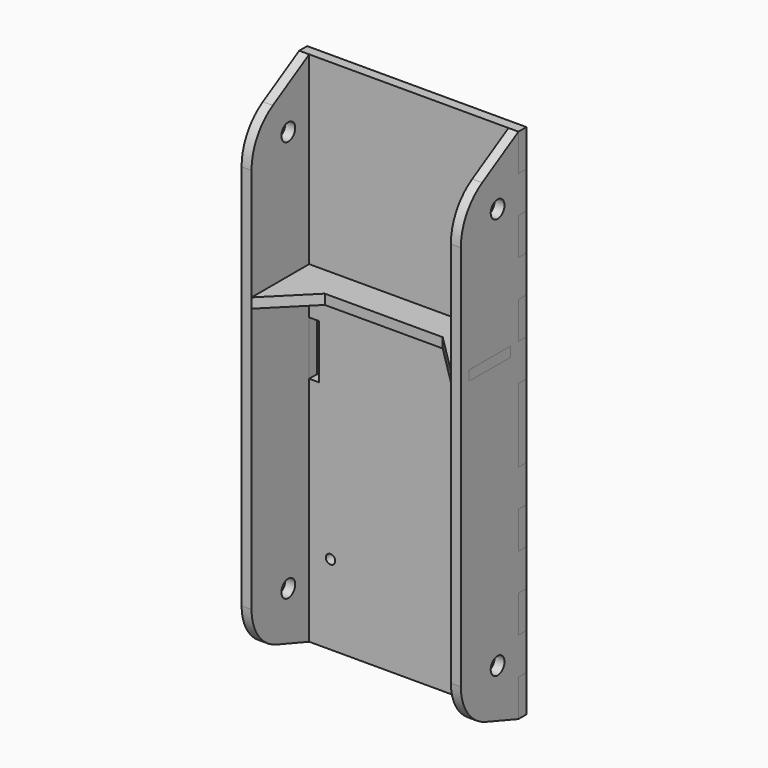
from build123d import *

# Parameters (mm, degrees)
F2_R     = 1.5
F2_W     = 3.175
F2_H     = 17.2357142857
F2_W_2   = 40
F2_H_2   = 3.175
F3_DEPTH = 3.175
F5_START = 31.825
F4_R     = 2.75
F4_W     = 16.65
F4_H     = 3.175
F5_DEPTH = 3.175
F8_DEPTH = 3.175


# Not quite as in the source:
# - a length typed as a fraction of an inch, garbled in the dataset ("3 / 203.2 mm" for 3/8 in), is restored


with BuildPart() as f3:
    # F2 (on Front) → F3 (new body)
    with BuildSketch(Plane.XZ):
        Polygon((-35, -25.4), (0, -25.4), (35, -25.4), (35, -13.6071428571), (31.825, -13.6071428571), (31.825, -1.8142857143), (35, -1.8142857143), (35, 9.9785714286), (31.825, 9.9785714286), (31.825, 21.7714285714), (35, 21.7714285714), (35, 33.5642857143), (31.825, 33.5642857143), (31.825, 45.3571428571), (35, 45.3571428571), (35, 57.15), (35, 68.9428571429), (31.825, 68.9428571429), (31.825, 80.7357142857), (35, 80.7357142857), (35, 92.5285714286), (31.825, 92.5285714286), (31.825, 104.3214285714), (35, 104.3214285714), (35, 116.1142857143), (31.825, 116.1142857143), (31.825, 127.9071428571), (35, 127.9071428571), (35, 139.7), (0, 139.7), (-35, 139.7), (-35, 127.9071428571), (-31.825, 127.9071428571), (-31.825, 116.1142857143), (-35, 116.1142857143), (-35, 104.3214285714), (-31.825, 104.3214285714), (-31.825, 92.5285714286), (-35, 92.5285714286), (-35, 80.7357142857), (-31.825, 80.7357142857), (-31.825, 68.9428571429), (-35, 68.9428571429), (-35, 57.15), (-35, 45.3571428571), (-31.825, 45.3571428571), (-31.825, 33.5642857143), (-35, 33.5642857143), (-35, 21.7714285714), (-31.825, 21.7714285714), (-31.825, 9.9785714286), (-35, 9.9785714286), (-35, -1.8142857143), (-31.825, -1.8142857143), (-31.825, -13.6071428571), (-35, -13.6071428571), align=None)
        with Locations((-25, 0)):
            Circle(F2_R, mode=Mode.SUBTRACT)
        with Locations((25, 0)):
            Circle(F2_R, mode=Mode.SUBTRACT)
        with Locations((-30.2375, 57.15)):
            Rectangle(F2_W, F2_H, mode=Mode.SUBTRACT)
        with Locations((0, 79.1482142857)):
            Rectangle(F2_W_2, F2_H_2, mode=Mode.SUBTRACT)
        with Locations((30.2375, 57.15)):
            Rectangle(F2_W, F2_H, mode=Mode.SUBTRACT)
    extrude(amount=F3_DEPTH)


with BuildPart() as f5:
    # F4 (on Right) → F5 (new body)
    with BuildSketch(Plane.YZ.offset(F5_START)):
        with BuildLine():
            Line((-16.2899039976, -20.8712812924), (-3.175, -25.4))
            Line((-3.175, -25.4), (-3.175, -13.6071428571))
            Line((-3.175, -13.6071428571), (0, -13.6071428571))
            Line((0, -13.6071428571), (0, -1.8142857143))
            Line((0, -1.8142857143), (-3.175, -1.8142857143))
            Line((-3.175, -1.8142857143), (-3.175, 9.9785714286))
            Line((-3.175, 9.9785714286), (0, 9.9785714286))
            Line((0, 9.9785714286), (0, 21.7714285714))
            Line((0, 21.7714285714), (-3.175, 21.7714285714))
            Line((-3.175, 21.7714285714), (-3.175, 33.5642857143))
            Line((-3.175, 33.5642857143), (0, 33.5642857143))
            Line((0, 33.5642857143), (0, 45.3571428571))
            Line((0, 45.3571428571), (-3.175, 45.3571428571))
            Line((-3.175, 45.3571428571), (-3.175, 57.15))
            Line((-3.175, 57.15), (-3.175, 68.9428571429))
            Line((-3.175, 68.9428571429), (0, 68.9428571429))
            Line((0, 68.9428571429), (0, 80.7357142857))
            Line((0, 80.7357142857), (-3.175, 80.7357142857))
            Line((-3.175, 80.7357142857), (-3.175, 92.5285714286))
            Line((-3.175, 92.5285714286), (0, 92.5285714286))
            Line((0, 92.5285714286), (0, 104.3214285714))
            Line((0, 104.3214285714), (-3.175, 104.3214285714))
            Line((-3.175, 104.3214285714), (-3.175, 116.1142857143))
            Line((-3.175, 116.1142857143), (0, 116.1142857143))
            Line((0, 116.1142857143), (0, 127.9071428571))
            Line((0, 127.9071428571), (-3.175, 127.9071428571))
            Line((-3.175, 127.9071428571), (-3.175, 139.7))
            Line((-3.175, 139.7), (-17.6680646356, 131.239778703))
            ThreePointArc((-17.6680646356, 131.239778703), (-23.8970296567, 124.9659809178), (-26.175, 116.4236513176))
            Line((-26.175, 116.4236513176), (-26.175, -7))
            ThreePointArc((-26.175, -7), (-23.4508883805, -15.5165657349), (-16.2899039976, -20.8712812924))
        make_face()
        with Locations((-11.5, -7)):
            Circle(F4_R, mode=Mode.SUBTRACT)
        with Locations((-14.675, 79.1482142857)):
            Rectangle(F4_W, F4_H, mode=Mode.SUBTRACT)
        with Locations((-11.5, 121.3)):
            Circle(F4_R, mode=Mode.SUBTRACT)
    extrude(amount=F5_DEPTH)


with BuildPart() as f6_1:
    # F6: instance of F5
    add(f5.part.mirror(Plane.YZ))


with BuildPart() as f8:
    # F7 (on face) → F8 (new body)
    with BuildSketch(Plane.XY.offset(77.5607142857)):
        Polygon((-18.825, -13.175), (0, -13.175), (18.825, -13.175), (31.825, -26.175), (31.825, -23), (35, -23), (35, -6.35), (31.825, -6.35), (31.825, -3.175), (20, -3.175), (20, 0), (0, 0), (-20, 0), (-20, -3.175), (-31.825, -3.175), (-31.825, -6.35), (-35, -6.35), (-35, -23), (-31.825, -23), (-31.825, -26.175), align=None)
    extrude(amount=F8_DEPTH)


solid = Compound([f3.part, f5.part, f6_1.part, f8.part])
